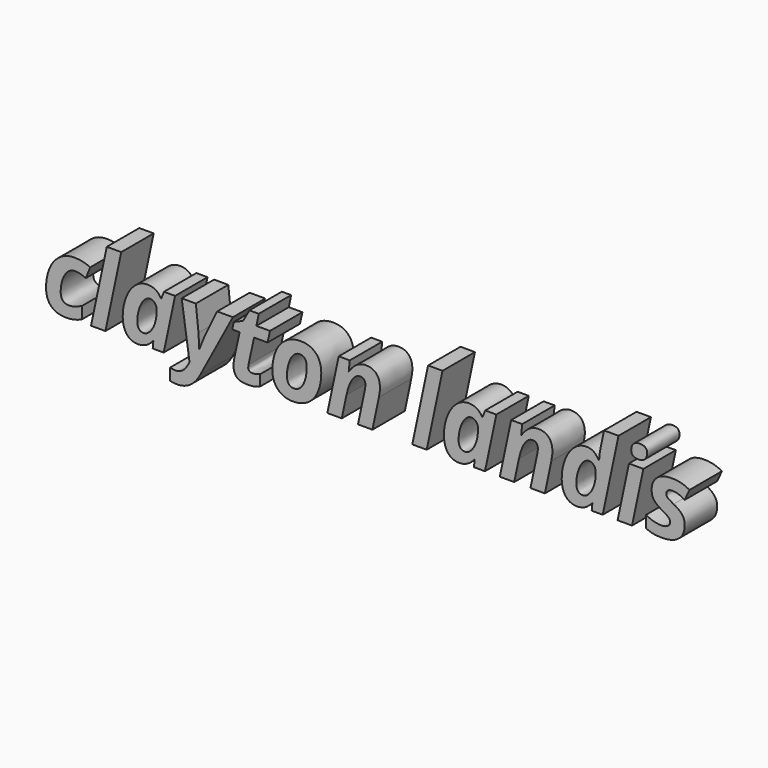
from build123d import *

# Parameters (mm, degrees)
F0_TEXT_SIZE = 61.5826600956
F1_DEPTH     = 25.4


# Not quite as in the source:
# - Text() gives the source's letters only with a copy of the font that has no kerning and outlines rounded to 1/6400 em; it was checked with that copy


with BuildPart() as f1:
    # F0 (on Front) → F1 (new body)
    with BuildSketch(Plane.XZ):
        with Locations((-213.621340692, 0)):
            Text('clayton landis', F0_TEXT_SIZE, font='Open Sans', font_style=FontStyle.BOLDITALIC, text_align=(TextAlign.LEFT, TextAlign.BOTTOM))
    extrude(amount=F1_DEPTH)


solid = f1.part
